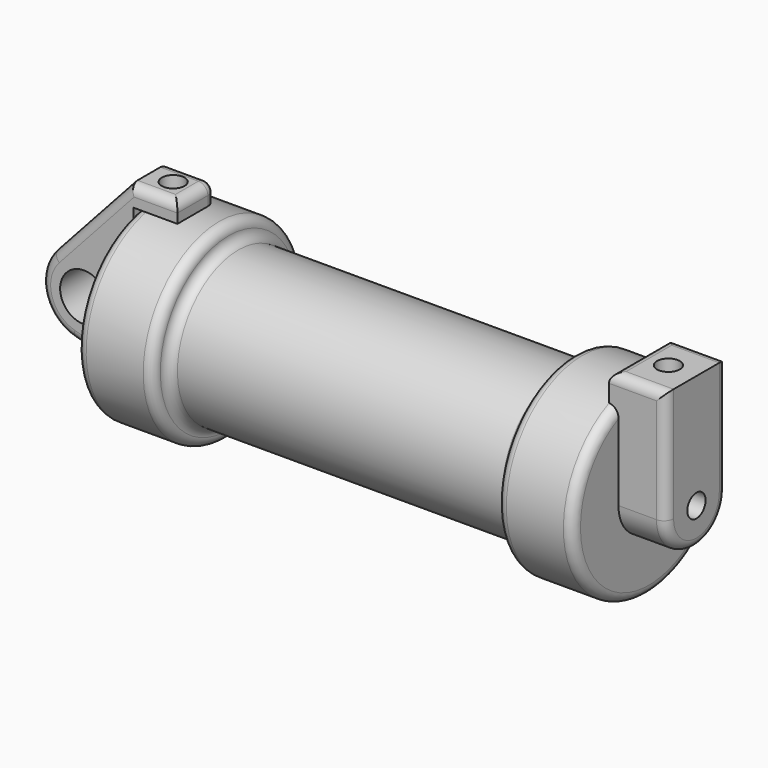
from build123d import *

# Parameters (mm, degrees)
F0_W      = 5.842
F0_H      = 12.7
F0_R      = 3.175
F2_DEPTH  = 3.175
F3_R      = 1.524
F4_DEPTH  = 6.35
F5_DEPTH  = 1.27
F6_DEPTH  = 56.134
F7_R      = 1.524
F9_DEPTH  = 17.78
F8_R      = 1.524
F10_DEPTH = 10.414
F11_R     = 1.26999
F11_2_R   = 1.26999


# Not quite as in the source:
# - a fillet or chamfer is up to 0.001 mm smaller than in the source, because OpenCascade refuses the exact size


with BuildPart() as f1:
    # F0 (on Front) → F1 (revolve)
    with BuildSketch(Plane.XZ):
        Polygon((5.842, 12.7), (5.842, 0), (66.294, 0), (66.294, 12.7), (56.134, 12.7), (56.134, 10.16), (10.16, 10.16), (10.16, 12.7), align=None)
        with Locations((2.921, 6.35)):
            Rectangle(F0_W, F0_H)
    revolve(axis=Axis((33.147, 0, 0), (-1, 0, 0)))

    # F3 (on face) → F4 (join)
    with BuildSketch(Plane.YZ.offset(66.294)):
        with BuildLine():
            ThreePointArc((-5.08, 0), (0, -5.08), (5.08, 0))
            ThreePointArc((5.08, 0), (0, 5.08), (-5.08, 0))
        make_face()
        Circle(F3_R, mode=Mode.SUBTRACT)
        with BuildLine():
            ThreePointArc((-5.08, 0), (0, 5.08), (5.08, 0))
            Line((5.08, 0), (5.08, 11.6397422652))
            ThreePointArc((5.08, 11.6397422652), (0, 12.7), (-5.08, 11.6397422652))
            Line((-5.08, 11.6397422652), (-5.08, 0))
        make_face()
        with BuildLine():
            ThreePointArc((-5.08, 11.6397422652), (0, 12.7), (5.08, 11.6397422652))
            Line((5.08, 11.6397422652), (5.08, 15.24))
            Line((5.08, 15.24), (-5.08, 15.24))
            Line((-5.08, 15.24), (-5.08, 11.6397422652))
        make_face()
    extrude(amount=F4_DEPTH)

    # F5 (add): a face of the model
    f5_faces = [f1.faces().sort_by_distance(p)[0] for p in [
        (66.294, 0, 13.7792682875),
    ]]
    extrude(f5_faces, amount=F5_DEPTH)

    # F6 (cut, through all): a face of the model
    f6_faces = [f1.faces().sort_by_distance(p)[0] for p in [
        (66.294, 0, 0),
    ]]
    extrude(f6_faces, amount=-F6_DEPTH, mode=Mode.SUBTRACT)

    # F8 (on face) → F10 (cut)
    with BuildSketch(Plane.XY.offset(15.24)):
        with Locations((68.834, 0.0751180435)):
            Circle(F8_R)
    extrude(amount=-F10_DEPTH, mode=Mode.SUBTRACT)

    # F11 (radius 1.27 in the source; OpenCascade refuses exactly that, so slightly less here)
    f11_edges = [f1.edges().sort_by_distance(p)[0] for p in [
        (68.834, 5.08, 15.24),
        (72.644, 5.08, 7.62),
        (68.834, -5.08, 15.24),
        (65.024, 0, 15.24),
        (66.294, 0, -12.7),
        (10.16, 0, -10.16),
        (0, 0, -12.7),
        (56.134, 0, -12.7),
        (56.134, 0, -10.16),
        (33.147, 0, 10.16),
        (10.16, 0, -12.7),
        (5.08, 0, 12.7),
        (72.644, -5.08, 7.62),
        (72.644, 0, -5.08),
    ]]
    fillet(f11_edges, radius=F11_R)


with BuildPart() as f2:
    # F0 (on Front) → F2 (new body, symmetric)
    with BuildSketch(Plane.XZ):
        with BuildLine():
            Line((-0.9398, 0), (0, 0))
            Line((0, 0), (0, 12.7))
            Line((0, 12.7), (5.842, 12.7))
            Line((5.842, 12.7), (5.842, 15.24))
            Line((5.842, 15.24), (-0.508, 15.24))
            Line((-0.508, 15.24), (-10.8806298187, 3.8475430269))
            ThreePointArc((-10.8806298187, 3.8475430269), (-4.5919612295, 5.3297205562), (-0.9398, 0))
        make_face()
        with BuildLine():
            ThreePointArc((-8.1826630726, -5.5069827884), (-3.1957909266, -4.5493385486), (-0.9398, 0))
            ThreePointArc((-0.9398, 0), (-4.5919612295, 5.3297205562), (-10.8806298187, 3.8475430269))
            ThreePointArc((-10.8806298187, 3.8475430269), (-12.1459778134, -1.5837270034), (-8.1826630726, -5.5069827884))
        make_face()
        with Locations((-6.6548, 0)):
            Circle(F0_R, mode=Mode.SUBTRACT)
        with BuildLine():
            Line((5.842, 0), (0, 0))
            Line((0, 0), (-0.9398, 0))
            ThreePointArc((-0.9398, 0), (-3.1957909266, -4.5493385486), (-8.1826630726, -5.5069827884))
            Line((-8.1826630726, -5.5069827884), (5.842, -9.398))
            Line((5.842, -9.398), (5.842, 0))
        make_face()
    extrude(amount=F2_DEPTH, both=True)

    # F7 (on face) → F9 (cut)
    with BuildSketch(Plane.XY.offset(15.24)):
        with Locations((2.5998465717, 0.1684235758)):
            Circle(F7_R)
    extrude(amount=-F9_DEPTH, mode=Mode.SUBTRACT)

    # F11#2 (radius 1.27 in the source; OpenCascade refuses exactly that, so slightly less here)
    f11_2_edges = [f2.edges().sort_by_distance(p)[0] for p in [
        (5.842, 3.175, 13.97),
        (2.667, 3.175, 15.24),
        (-1.170332, 3.175, -7.452491),
        (-8.182663, 0, -5.506983),
        (5.842, 0, -9.398),
        (-1.170332, -3.175, -7.452491),
        (2.667, -3.175, 15.24),
        (5.842, 0, 15.24),
        (-5.694315, 3.175, 9.543772),
        (-12.145978, 3.175, -1.583727),
        (-5.694315, -3.175, 9.543772),
        (-12.145978, -3.175, -1.583727),
    ]]
    fillet(f11_2_edges, radius=F11_2_R)


solid = Compound([f1.part, f2.part])
